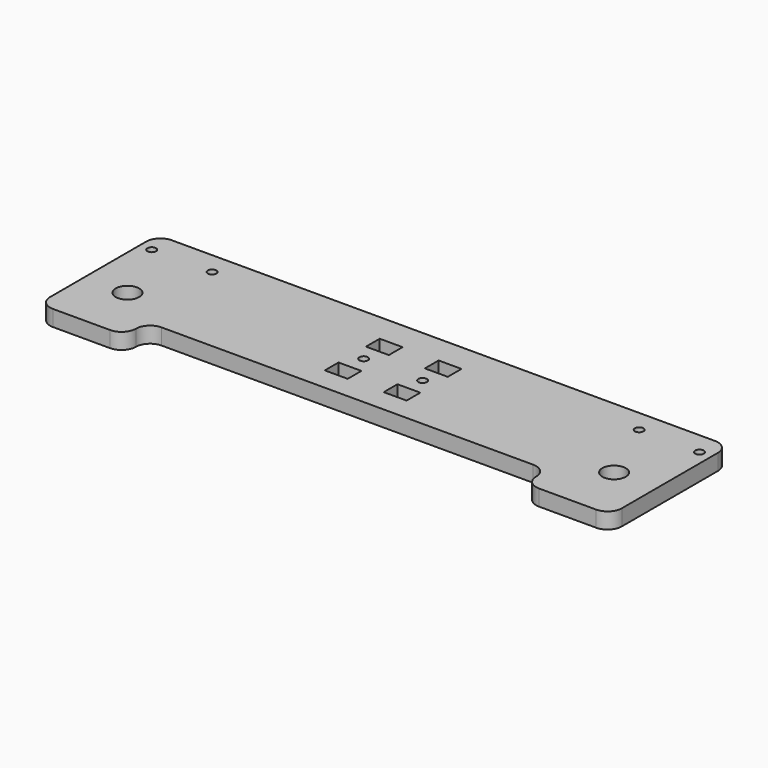
from build123d import *

# Parameters (mm, degrees)
F0_W     = 200
F0_H     = 52
F0_R     = 4.1
F0_W_2   = 8
F0_H_2   = 6
F0_R_2   = 1.5
F1_DEPTH = 5.588
F2_W     = 140
F2_H     = 10
F3_DEPTH = 25
F4_R     = 4.99999


# Not quite as in the source:
# - a fillet or chamfer is up to 0.001 mm smaller than in the source, because OpenCascade refuses the exact size


with BuildPart() as f1:
    # F0 (on Top) → F1 (new body)
    with BuildSketch(Plane.XY):
        Rectangle(F0_W, F0_H)
        with Locations((-85.1, -5.8)):
            Circle(F0_R, mode=Mode.SUBTRACT)
        with Locations((-10.3, -5)):
            Rectangle(F0_W_2, F0_H_2, mode=Mode.SUBTRACT)
        with Locations((10.3, -5)):
            Rectangle(F0_W_2, F0_H_2, mode=Mode.SUBTRACT)
        with Locations((85.1, -5.8)):
            Circle(F0_R, mode=Mode.SUBTRACT)
        with Locations((-10.3, 4)):
            Circle(F0_R_2, mode=Mode.SUBTRACT)
        with Locations((-95.8, 18.2)):
            Circle(F0_R_2, mode=Mode.SUBTRACT)
        with Locations((-74.7, 18.2)):
            Circle(F0_R_2, mode=Mode.SUBTRACT)
        with Locations((-10.3, 13)):
            Rectangle(F0_W_2, F0_H_2, mode=Mode.SUBTRACT)
        with Locations((10.3, 4)):
            Circle(F0_R_2, mode=Mode.SUBTRACT)
        with Locations((10.3, 13)):
            Rectangle(F0_W_2, F0_H_2, mode=Mode.SUBTRACT)
        with Locations((74.7, 18.2)):
            Circle(F0_R_2, mode=Mode.SUBTRACT)
        with Locations((95.8, 18.2)):
            Circle(F0_R_2, mode=Mode.SUBTRACT)
    extrude(amount=F1_DEPTH)

    # F2 (on face) → F3 (cut)
    with BuildSketch(Plane.XY.offset(5.588)):
        with Locations((0, -21)):
            Rectangle(F2_W, F2_H)
    extrude(amount=-F3_DEPTH, mode=Mode.SUBTRACT)

    # F4 (radius 5 in the source; OpenCascade refuses exactly that, so slightly less here)
    f4_edges = [f1.edges().sort_by_distance(p)[0] for p in [
        (-100, 26, 2.794),
        (-100, -26, 2.794),
        (-70, -26, 2.794),
        (-70, -16, 2.794),
        (70, -16, 2.794),
        (70, -26, 2.794),
        (100, -26, 2.794),
        (100, 26, 2.794),
    ]]
    fillet(f4_edges, radius=F4_R)


solid = f1.part
